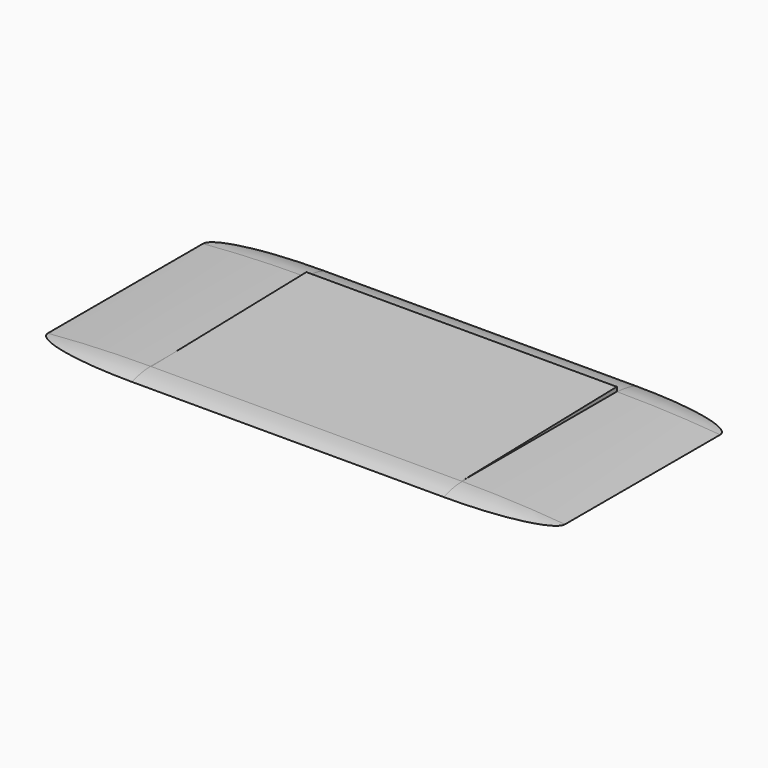
from build123d import *

# Parameters (mm, degrees)
F0_W         = 120
F0_H         = 75
F1_DEPTH     = 1
F0_W_2       = 24
F0_H_2       = 45
F2_DEPTH     = 2
F3_DEPTH     = 2
F4_DEPTH     = 2
F6_DEPTH     = 1000
F7_T1_DEPTH  = 194.2686044191
F8_T1_DEPTH  = 194.2686044191
F9_T1_DEPTH  = 72.2925582324
F9_T4_ANGLE  = 12.3400437426
F9_T6_ANGLE  = 12.3400437426
F10_T1_DEPTH = 72.2925582324
F10_T4_ANGLE = 12.3400437426
F10_T6_ANGLE = 12.3400437426


# Not quite as in the source:
# - a fillet or chamfer that OpenCascade refuses, or shapes differently, is made with other operations: its cross-section is extruded or revolved along the edge and cut away or added


with BuildPart() as f1:
    # F0 (on Top) → F1 (new body)
    with BuildSketch(Plane.XY):
        Rectangle(F0_W, F0_H)
        Polygon((-36, -22.5), (-36, 22.5), (-12, 22.5), (12, 22.5), (36, 22.5), (36, -22.5), (12, -22.5), (-12, -22.5), align=None, mode=Mode.SUBTRACT)
    extrude(amount=F1_DEPTH)

    # F0 (on Top) → F2 (join)
    with BuildSketch(Plane.XY):
        with Locations((-24, 0)):
            Rectangle(F0_W_2, F0_H_2)
    extrude(amount=F2_DEPTH)

    # F0 (on Top) → F3 (join)
    with BuildSketch(Plane.XY):
        Rectangle(F0_W_2, F0_H_2)
    extrude(amount=F3_DEPTH)

    # F0 (on Top) → F4 (join)
    with BuildSketch(Plane.XY):
        with Locations((24, 0)):
            Rectangle(F0_W_2, F0_H_2)
    extrude(amount=F4_DEPTH)

    # F5 (on face) → F6 (cut)
    with BuildSketch(Plane(origin=(-60, 0, 0), x_dir=(0, -1, 0), z_dir=(-1, 0, 0))):
        Polygon((22.5, 2), (-22.5, 2), (22.5, 1), align=None)
    extrude(amount=-F6_DEPTH, mode=Mode.SUBTRACT)

    # F7: fillet of radius 285 on 1 edges, made by hand

    # F7_s2 → F7_t1 (cut)
    with BuildSketch(Plane.XZ.offset(-97.1343022095)):
        with BuildLine():
            ThreePointArc((-36.1462791162, 1), (-48.0836155025, 0.7498902546), (-60, 0))
            Line((-60, 0), (-60, 1))
            Line((-60, 1), (-36.1462791162, 1))
        make_face()
    extrude(amount=F7_T1_DEPTH, mode=Mode.SUBTRACT)

    # F8: fillet of radius 285 on 1 edges, made by hand

    # F8_s2 → F8_t1 (cut)
    with BuildSketch(Plane.XZ.offset(-97.1343022095)):
        with BuildLine():
            ThreePointArc((36.1462791162, 1), (48.0836155025, 0.7498902546), (60, 0))
            Line((60, 0), (60, 1))
            Line((60, 1), (36.1462791162, 1))
        make_face()
    extrude(amount=F8_T1_DEPTH, mode=Mode.SUBTRACT)

    # F9: fillet of radius 15 on 1 edges, made by hand

    # F9_s2 → F9_t1 (cut)
    with BuildSketch(Plane.YZ.offset(-36.1462791162)):
        with BuildLine():
            ThreePointArc((-22.5, 1), (-33.1066017178, -3.3933982822), (-37.5, -14))
            Line((-37.5, -14), (-37.5, 1))
            Line((-37.5, 1), (-22.5, 1))
        make_face()
    extrude(amount=F9_T1_DEPTH, mode=Mode.SUBTRACT)

    # F9_s3 → F9_t4 (revolve, cut)
    with BuildSketch(Plane(origin=(-93.7876438564, 0, -20.5176876571), x_dir=(0, 1, 0), z_dir=(-0.9768964499, 0, -0.2137131866))):
        with BuildLine():
            ThreePointArc((-22.5, -15.2863447158), (-33.1066017178, -10.8929464336), (-37.5, -0.2863447158))
            Line((-37.5, -0.2863447158), (-37.5, -15.2863447158))
            Line((-37.5, -15.2863447158), (-22.5, -15.2863447158))
        make_face()
    revolve(axis=Axis((-36.1462791167, -37.5, -283.9999999893), (0, 1, 0)), revolution_arc=F9_T4_ANGLE, mode=Mode.SUBTRACT)

    # F9_s5 → F9_t6 (revolve, cut)
    with BuildSketch(Plane.YZ.offset(36.1462791167)):
        with BuildLine():
            ThreePointArc((-22.5, 1), (-33.1066017178, -3.3933982822), (-37.5, -14))
            Line((-37.5, -14), (-37.5, 1))
            Line((-37.5, 1), (-22.5, 1))
        make_face()
    revolve(axis=Axis((36.1462791167, -37.5, -283.9999999893), (0, 1, 0)), revolution_arc=F9_T6_ANGLE, mode=Mode.SUBTRACT)

    # F10: fillet of radius 15 on 1 edges, made by hand

    # F10_s2 → F10_t1 (cut)
    with BuildSketch(Plane.YZ.offset(-36.1462791162)):
        with BuildLine():
            ThreePointArc((37.5, -14), (33.1066017178, -3.3933982822), (22.5, 1))
            Line((22.5, 1), (37.5, 1))
            Line((37.5, 1), (37.5, -14))
        make_face()
    extrude(amount=F10_T1_DEPTH, mode=Mode.SUBTRACT)

    # F10_s3 → F10_t4 (revolve, cut)
    with BuildSketch(Plane.YZ.offset(36.1462791167)):
        with BuildLine():
            ThreePointArc((37.5, -14), (33.1066017178, -3.3933982822), (22.5, 1))
            Line((22.5, 1), (37.5, 1))
            Line((37.5, 1), (37.5, -14))
        make_face()
    revolve(axis=Axis((36.1462791167, 37.5, -283.9999999893), (0, 1, 0)), revolution_arc=F10_T4_ANGLE, mode=Mode.SUBTRACT)

    # F10_s5 → F10_t6 (revolve, cut)
    with BuildSketch(Plane(origin=(-93.7876438564, 0, -20.5176876571), x_dir=(0, 1, 0), z_dir=(-0.9768964499, 0, -0.2137131866))):
        with BuildLine():
            ThreePointArc((37.5, -0.2863447158), (33.1066017178, -10.8929464336), (22.5, -15.2863447158))
            Line((22.5, -15.2863447158), (37.5, -15.2863447158))
            Line((37.5, -15.2863447158), (37.5, -0.2863447158))
        make_face()
    revolve(axis=Axis((-36.1462791167, 37.5, -283.9999999893), (0, 1, 0)), revolution_arc=F10_T6_ANGLE, mode=Mode.SUBTRACT)


solid = f1.part
